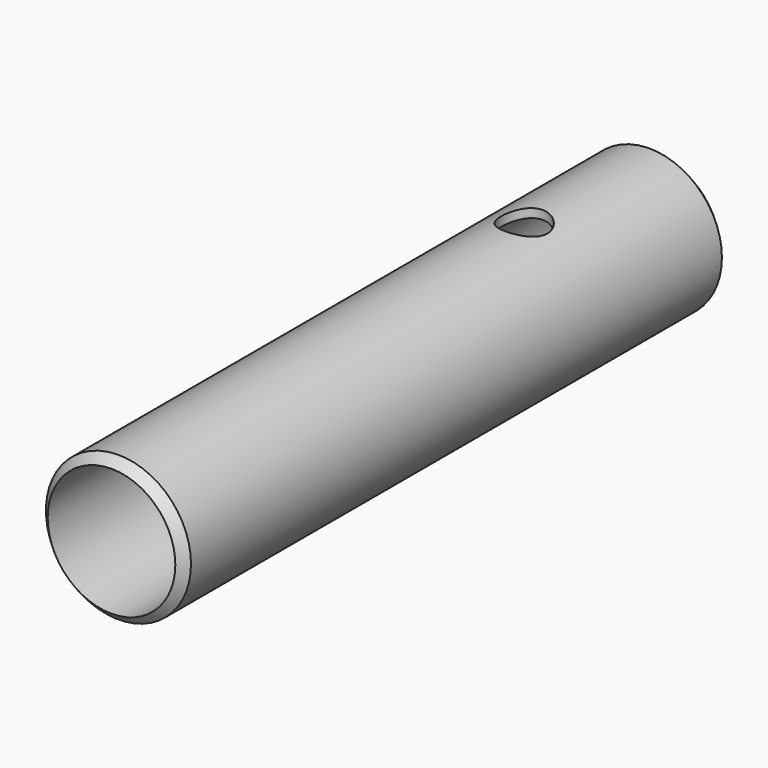
from build123d import *

# Parameters (mm, degrees)
F0_R     = 7.9375
F1_DEPTH = 76.2
F3_D     = 13.97
F3_DEPTH = 76.2
F3_TIP   = 4.1970114239
F7_D     = 5.08
F7_DEPTH = 25.4
F7_TIP   = 1.5261859723


# Not quite as in the source:
# - a fillet or chamfer that OpenCascade refuses, or shapes differently, is made with other operations: its cross-section is extruded or revolved along the edge and cut away or added


with BuildPart() as f1:
    # F0 (on Front) → F1 (new body)
    with BuildSketch(Plane.XZ):
        Circle(F0_R)
    extrude(amount=F1_DEPTH)

    # F3
    with Locations(Plane(origin=(0, 0, 0), x_dir=(1, 0, 0), z_dir=(0, 1, 0))):
        with Locations((0, 0)):
            Hole(F3_D / 2, depth=F3_DEPTH)
            with Locations((0, 0, -(F3_DEPTH + F3_TIP / 2))):  # 118° drill point
                Cone(0, F3_D / 2, F3_TIP, mode=Mode.SUBTRACT)

    # F4: chamfer of 1.778 on 1 edges, made by hand

    # F4_s1 → F4_t2 (revolve, cut)
    with BuildSketch(Plane.XY):
        Polygon((7.9375, -74.422), (6.1595, -76.2), (7.9375, -76.2), align=None)
    revolve(axis=Axis((0, -76.2, 0), (0, -1, 0)), mode=Mode.SUBTRACT)

    # F5: chamfer of 1.778 on 1 edges, made by hand

    # F5_s1 → F5_t2 (revolve, cut)
    with BuildSketch(Plane.XY):
        Polygon((7.9375, -1.778), (6.1595, 0), (7.9375, 0), align=None)
    revolve(axis=Axis((0, 0, 0), (0, -1, 0)), mode=Mode.SUBTRACT)

    # F7 (one way)
    with BuildSketch(Plane(origin=(0, 0, 0), x_dir=(1, 0, 0), z_dir=(0, 0, -1))):
        with Locations((0, 18.9180281013)):
            Circle(F7_D / 2)
    extrude(amount=-F7_DEPTH, mode=Mode.SUBTRACT)
    with Locations(Plane(origin=(0, 0, 0), x_dir=(1, 0, 0), z_dir=(0, 0, -1))):
        with Locations((0, 18.9180281013)):
            with Locations((0, 0, -(F7_DEPTH + F7_TIP / 2))):  # 118° drill point
                Cone(0, F7_D / 2, F7_TIP, mode=Mode.SUBTRACT)


solid = f1.part
